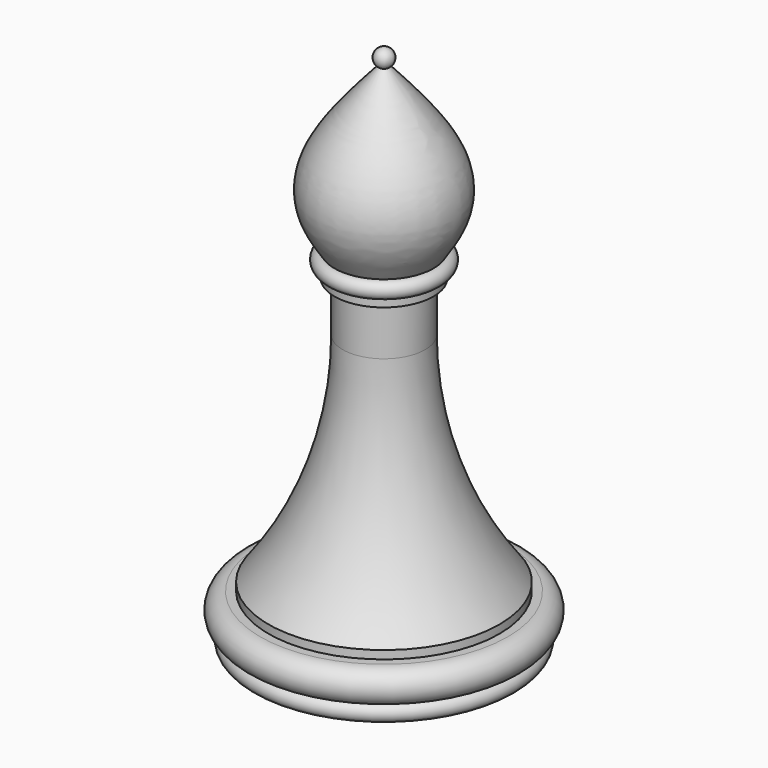
from build123d import *

# Parameters (mm, degrees)
F4_DEPTH = 37.846


# Not quite as in the source:
# - the dataset's text gives a spline's control points without its knots; the knots are read off the source's solid


with BuildPart() as f1:
    # F0 (on Front) → F1 (revolve)
    with BuildSketch(Plane.XZ):
        with BuildLine():
            Line((0.8687140835, -0.0766073585), (19.9186500873, -0.0272287397))
            ThreePointArc((19.9186500873, -0.0272287397), (21.2238316031, 1.1144988687), (20.2733522924, 2.5648884029))
            ThreePointArc((20.2733522924, 2.5648884029), (20.272604442, 2.5647830482), (20.2718565603, 2.5646779158))
            ThreePointArc((20.2718565603, 2.5646779158), (20.270477887, 2.564484705), (20.269099108, 2.5642922499))
            ThreePointArc((20.269099108, 2.5642922499), (20.0942950627, 2.5460803401), (19.9186500873, 2.54))
            Line((19.9186500873, 2.54), (0.868714004, 2.54))
            Line((0.868714004, 2.54), (0.8687140835, 0))
            Line((0.8687140835, 0), (0.8687140835, -0.0766073585))
        make_face()
        with BuildLine():
            ThreePointArc((20.2718565603, 2.5646779158), (20.272604442, 2.5647830482), (20.2733522924, 2.5648884029))
            ThreePointArc((20.2733522924, 2.5648884029), (22.4524203469, 5.2577871528), (19.9186500873, 7.62))
            Line((19.9186500873, 7.62), (18.6486500873, 7.62))
            Line((18.6486500873, 7.62), (0.8687138451, 7.62))
            Line((0.8687138451, 7.62), (0.868714004, 2.54))
            Line((0.868714004, 2.54), (19.9186500873, 2.54))
            ThreePointArc((19.9186500873, 2.54), (20.0942950627, 2.5460803401), (20.269099108, 2.5642922499))
            ThreePointArc((20.269099108, 2.5642922499), (20.270477887, 2.564484705), (20.2718565603, 2.5646779158))
        make_face()
        with BuildLine():
            Line((0.8687138451, 7.62), (18.6486500873, 7.62))
            Line((18.6486500873, 7.62), (18.6486500873, 8.89))
            ThreePointArc((18.6486500873, 8.89), (10.1548470737, 24.6914739709), (7.2187125191, 42.3892247649))
            Line((7.2187125191, 42.3892247649), (7.2187125191, 50.0092247649))
            Line((7.2187125191, 50.0092247649), (0.8687125191, 50.0092245663))
            Line((0.8687125191, 50.0092245663), (0.8687138451, 7.62))
        make_face()
        Polygon((0.8687124794, 51.2792245663), (0.8687125191, 50.0092245663), (7.2187125191, 50.0092247649), (8.4887125191, 50.0092248046), (8.4887124794, 51.2792248046), align=None)
        with BuildLine():
            Line((0.8687123999, 53.8192245663), (0.8687124794, 51.2792245663))
            Line((0.8687124794, 51.2792245663), (8.4887124794, 51.2792248046))
            ThreePointArc((8.4887124794, 51.2792248046), (9.7587124397, 52.5492248444), (8.4887123999, 53.8192248046))
            Line((8.4887123999, 53.8192248046), (0.8687123999, 53.8192245663))
        make_face()
        with BuildLine():
            Line((0.8687116198, 78.7601301898), (0.8687123999, 53.8192245663))
            Line((0.8687123999, 53.8192245663), (8.4887123999, 53.8192248046))
            add(Edge.make_bspline(
                [(1.6365837319, 78.7601301898), (5.4186590488, 74.5149174819), (11.8101021821, 67.3254379274), (11.9301625008, 59.0236863072), (9.5969562369, 55.4949238027), (8.4887123999, 53.8192248046)],
                knots=[0, 0, 0, 0, 0.4323934447, 0.7302637057, 1, 1, 1, 1], degree=3))
            Line((1.6365837319, 78.7601301898), (0.8687115409, 78.7601301898))
        make_face()
        with BuildLine():
            Line((0.8687115409, 81.28), (0.8687116198, 78.7601301898))
            Line((0.8687115409, 78.7601301898), (1.6365837319, 78.7601301898))
            ThreePointArc((1.6365837319, 78.7601301898), (2.1986220113, 80.3083289619), (0.8687115409, 81.28))
        make_face()
    revolve(axis=Axis((0.8687128122, 0, 40.64), (-3.13e-08, 0, 1)))

    # F3 (on offset) → F4 (cut)
    with BuildSketch(Plane.XY.offset(98.552)):
        with BuildLine():
            add(Edge.make_bspline(
                [(-0.8870822494, 11.3366749138), (-0.2147011578, 9.1421833591), (1.1349142574, 4.7373604577), (-3.668479662, -1.8981738182), (-8.377801508, -1.2887326345), (-10.7270758599, -0.9847091278)],
                knots=[0, 0, 0, 0, 0.3322437722, 0.6668856726, 1, 1, 1, 1], degree=3))
            Line((-0.8870822494, 11.3366749138), (-3.5585010522, 10.5181657302))
            add(Edge.make_bspline(
                [(-3.5585010522, 10.5181657302), (-3.3055312646, 9.692532664), (-2.9566781524, 8.5406032849), (-2.6979877827, 7.2079674881), (-2.6362155672, 6.4694176926), (-2.6484361925, 5.9315025918), (-2.6885550798, 5.5485331656), (-2.759454646, 5.1842243218), (-2.8716568974, 4.7969109038), (-3.0245694503, 4.3987727881), (-3.2794968699, 3.8666639521), (-3.684944703, 3.2243750018), (-4.1697737375, 2.6723602253), (-4.5747953406, 2.3132410275), (-4.8780925155, 2.0898453689), (-5.1716732115, 1.9155559626), (-5.4465299214, 1.7895913286), (-5.7568599619, 1.6844232462), (-6.2208776696, 1.575597816), (-6.9139940857, 1.4996766218), (-8.2595367302, 1.5180233246), (-9.4869328126, 1.6721007861), (-10.3684898932, 1.7861845562)],
                knots=[0, 0, 0, 0, 0.125, 0.1875, 0.25, 0.28125, 0.3125, 0.34375, 0.375, 0.40625, 0.4375, 0.5, 0.5625, 0.59375, 0.625, 0.65625, 0.6875, 0.71875, 0.75, 0.8125, 0.875, 1, 1, 1, 1], degree=3))
            Line((-10.3684898932, 1.7861845562), (-10.7270758599, -0.9847091278))
        make_face()
    extrude(amount=-F4_DEPTH, mode=Mode.SUBTRACT)


solid = f1.part
